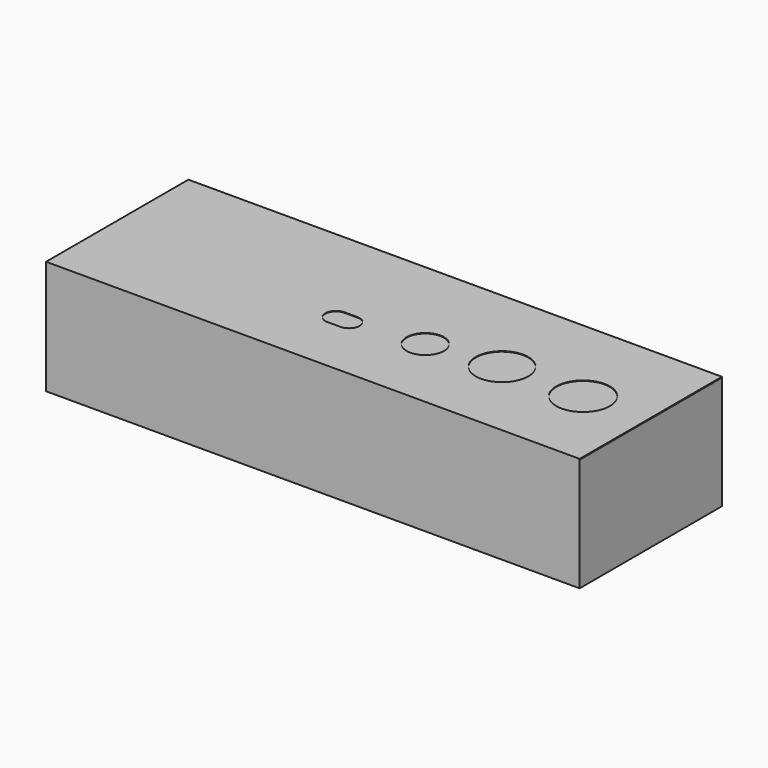
from build123d import *

# Parameters (mm, degrees)
F1_DEPTH = 209.55
F3_DEPTH = 0.4064


# Not quite as in the source:
# - the dataset's text gives a spline's control points without its knots; the knots are read off the source's solid


with BuildPart() as f1:
    # F0 (on Right) → F1 (new body, symmetric)
    with BuildSketch(Plane.YZ):
        Polygon((-139.7, 0), (0, 0), (0, 88.9), (-139.2936, 88.9), (-139.2936, 89.154), (0, 89.154), (0, 89.5604), (-139.7, 89.5604), align=None)
    extrude(amount=F1_DEPTH, both=True)

    # F2 (on face) → F3 (cut, through all)
    with BuildSketch(Plane.XY.offset(89.5604)):
        with BuildLine():
            add(Edge.make_bspline(
                [(-30.6699001032, -91.9856678392), (-29.1271803032, -93.5287178392), (-26.9585029032, -94.4268618392), (-24.7768207032, -94.4268618392)],
                knots=[3, 3, 3, 3, 4, 4, 4, 4], degree=3))
            Line((-24.7768207032, -94.4268618392), (-14.4580707032, -94.4268618392))
            add(Edge.make_bspline(
                [(-14.4580707032, -94.4268618392), (-12.2754995032, -94.4268618392), (-10.1075587032, -93.5287178392), (-8.5648643032, -91.9856678392)],
                knots=[0, 0, 0, 0, 1, 1, 1, 1], degree=3))
            add(Edge.make_bspline(
                [(-8.5648643032, -91.9856678392), (-7.0217127032, -90.4429226392), (-6.1236703032, -88.2745754392), (-6.1236703032, -86.0924868392), (-6.1236703032, -83.9103220392), (-7.0217127032, -81.7420256392), (-8.5648643032, -80.1989248392)],
                knots=[1, 1, 1, 1, 2, 2, 2, 3, 3, 3, 3], degree=3))
            add(Edge.make_bspline(
                [(-8.5648643032, -80.1989248392), (-10.1075587032, -78.6562304392), (-12.2754995032, -77.7581118392), (-14.4580707032, -77.7581118392)],
                knots=[3, 3, 3, 3, 4, 4, 4, 4], degree=3))
            Line((-14.4580707032, -77.7581118392), (-24.7768207032, -77.7581118392))
            add(Edge.make_bspline(
                [(-24.7768207032, -77.7581118392), (-26.9585029032, -77.7581118392), (-29.1271803032, -78.6562304392), (-30.6699001032, -80.1989248392)],
                knots=[0, 0, 0, 0, 1, 1, 1, 1], degree=3))
            add(Edge.make_bspline(
                [(-30.6699001032, -80.1989248392), (-32.2126199032, -81.7420256392), (-33.1111957032, -83.9103220392), (-33.1111957032, -86.0924868392), (-33.1111957032, -88.2745754392), (-32.2126199032, -90.4429226392), (-30.6699001032, -91.9856678392)],
                knots=[1, 1, 1, 1, 2, 2, 2, 3, 3, 3, 3], degree=3))
        make_face()
        with BuildLine():
            add(Edge.make_bspline(
                [(50.7387254968, -69.3589668392), (48.0202142968, -66.6407604392), (44.1992668968, -65.0581118392), (40.3547990968, -65.0581118392)],
                knots=[7, 7, 7, 7, 8, 8, 8, 8], degree=3))
            add(Edge.make_bspline(
                [(40.3547990968, -65.0581118392), (36.5108392968, -65.0581118392), (32.6898918968, -66.6407604392), (29.9713806968, -69.3589668392)],
                knots=[0, 0, 0, 0, 1, 1, 1, 1], degree=3))
            add(Edge.make_bspline(
                [(29.9713806968, -69.3589668392), (27.2531742968, -72.0774526392), (25.6704240968, -75.8984254392), (25.6704240968, -79.7424868392), (25.6704240968, -83.5868276392), (27.2531742968, -87.4076226392), (29.9713806968, -90.1256512392)],
                knots=[1, 1, 1, 1, 2, 2, 2, 3, 3, 3, 3], degree=3))
            add(Edge.make_bspline(
                [(29.9713806968, -90.1256512392), (32.6898918968, -92.8441878392), (36.5108392968, -94.4268618392), (40.3547990968, -94.4268618392), (44.1992668968, -94.4268618392), (48.0202142968, -92.8441878392), (50.7387254968, -90.1256512392)],
                knots=[3, 3, 3, 3, 4, 4, 4, 5, 5, 5, 5], degree=3))
            add(Edge.make_bspline(
                [(50.7387254968, -90.1256512392), (53.4569318968, -87.4076226392), (55.0391740968, -83.5868276392), (55.0391740968, -79.7424868392), (55.0391740968, -75.8984254392), (53.4569318968, -72.0774526392), (50.7387254968, -69.3589668392)],
                knots=[5, 5, 5, 5, 6, 6, 6, 7, 7, 7, 7], degree=3))
        make_face()
        with BuildLine():
            add(Edge.make_bspline(
                [(110.4663682968, -59.1962744392), (106.6457510968, -55.3760128392), (101.2762418968, -53.1516840392), (95.8732046968, -53.1516840392)],
                knots=[7, 7, 7, 7, 8, 8, 8, 8], degree=3))
            add(Edge.make_bspline(
                [(95.8732046968, -53.1516840392), (90.4710310968, -53.1516840392), (85.1011662968, -55.3760128392), (81.2809046968, -59.1962744392)],
                knots=[0, 0, 0, 0, 1, 1, 1, 1], degree=3))
            add(Edge.make_bspline(
                [(81.2809046968, -59.1962744392), (77.4602620968, -63.0168662392), (75.2357046968, -68.3864262392), (75.2357046968, -73.7891840392), (75.2357046968, -79.1919418392), (77.4602620968, -84.5619844392), (81.2809046968, -88.3822460392)],
                knots=[1, 1, 1, 1, 2, 2, 2, 3, 3, 3, 3], degree=3))
            add(Edge.make_bspline(
                [(81.2809046968, -88.3822460392), (85.1011662968, -92.2026854392), (90.4710310968, -94.4266840392), (95.8732046968, -94.4266840392), (101.2762418968, -94.4266840392), (106.6457510968, -92.2026854392), (110.4663682968, -88.3822460392)],
                knots=[3, 3, 3, 3, 4, 4, 4, 5, 5, 5, 5], degree=3))
            add(Edge.make_bspline(
                [(110.4663682968, -88.3822460392), (114.2866298968, -84.5619844392), (116.5107046968, -79.1919418392), (116.5107046968, -73.7891840392), (116.5107046968, -68.3864262392), (114.2866298968, -63.0168662392), (110.4663682968, -59.1962744392)],
                knots=[5, 5, 5, 5, 6, 6, 6, 7, 7, 7, 7], degree=3))
        make_face()
        with BuildLine():
            add(Edge.make_bspline(
                [(174.0707622968, -58.5189326392), (170.1766628968, -54.6249856392), (164.7038772968, -52.3579340392), (159.1969032968, -52.3579340392)],
                knots=[7, 7, 7, 7, 8, 8, 8, 8], degree=3))
            add(Edge.make_bspline(
                [(159.1969032968, -52.3579340392), (153.6906150968, -52.3579340392), (148.2173722968, -54.6249856392), (144.3237300968, -58.5189326392)],
                knots=[0, 0, 0, 0, 1, 1, 1, 1], degree=3))
            add(Edge.make_bspline(
                [(144.3237300968, -58.5189326392), (140.4297322968, -62.4129304392), (138.1624266968, -67.8854620392), (138.1624266968, -73.3923090392), (138.1624266968, -78.8991306392), (140.4297322968, -84.3721448392), (144.3237300968, -88.2661426392), (148.2173722968, -92.1597848392), (153.6906150968, -94.4266840392), (159.1969032968, -94.4266840392), (164.7038772968, -94.4266840392), (170.1766628968, -92.1597848392), (174.0707622968, -88.2661426392)],
                knots=[1, 1, 1, 1, 2, 2, 2, 3, 3, 3, 4, 4, 4, 5, 5, 5, 5], degree=3))
            add(Edge.make_bspline(
                [(174.0707622968, -88.2661426392), (177.9644044968, -84.3721448392), (180.2312782968, -78.8991306392), (180.2312782968, -73.3923090392), (180.2312782968, -67.8854620392), (177.9644044968, -62.4129304392), (174.0707622968, -58.5189326392)],
                knots=[5, 5, 5, 5, 6, 6, 6, 7, 7, 7, 7], degree=3))
        make_face()
    extrude(amount=-F3_DEPTH, mode=Mode.SUBTRACT)


solid = f1.part
